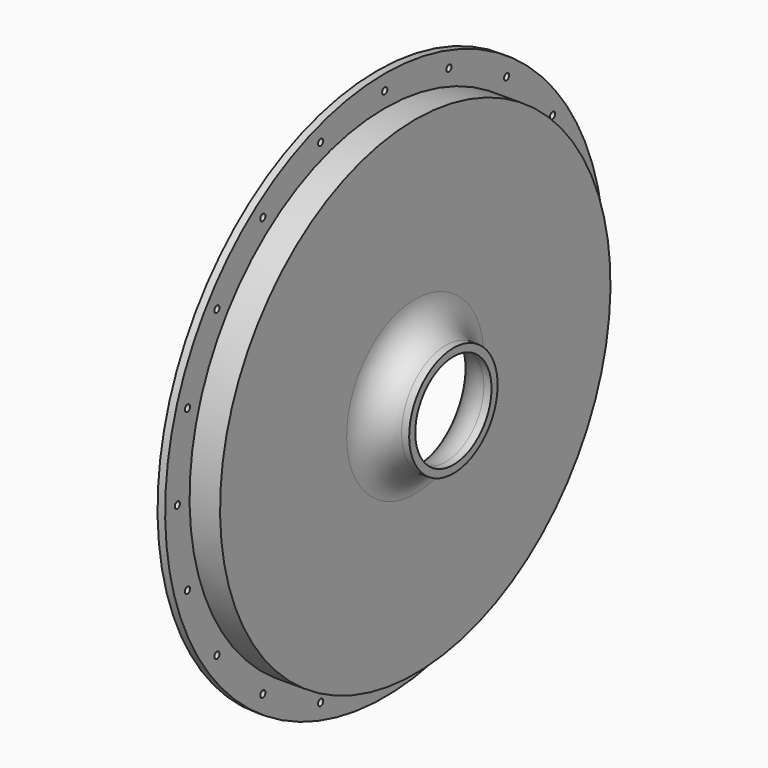
from build123d import *

# Parameters (mm, degrees)
F3_D            = 8.5
F3_COPIES_COUNT = 20


# Not quite as in the source:
# - a pattern or mirror of a feature is missing from the dataset's text; its kind, count and spacing are read off the source's solid


with BuildPart() as f1:
    # F0 (on Front) → F1 (revolve)
    with BuildSketch(Plane.XZ):
        with BuildLine():
            Line((40, 310), (40, 112.5))
            ThreePointArc((40, 112.5), (54.6446609407, 77.1446609407), (90, 62.5))
            Line((90, 62.5), (100, 62.5))
            Line((100, 62.5), (100, 72.5))
            Line((100, 72.5), (90, 72.5))
            ThreePointArc((90, 72.5), (61.7157287525, 84.2157287525), (50, 112.5))
            Line((50, 112.5), (50, 320))
            Line((50, 320), (10, 320))
            Line((10, 320), (10, 360))
            Line((10, 360), (0, 360))
            Line((0, 360), (0, 310))
            Line((0, 310), (40, 310))
        make_face()
    revolve(axis=Axis((50, 0, 0), (1, 0, 0)))

    # F3 (through all)
    with Locations(Plane.YZ.offset(10)):
        with Locations((0, 340)):
            f3 = Hole(F3_D / 2)

    # F3_copies: F3 ×20 about axis
    f3_copies_axis = Axis((0, 0, 0), (1, 0, 0))
    for i in range(1, F3_COPIES_COUNT):
        add(f3.rotate(f3_copies_axis, i * 360 / F3_COPIES_COUNT), mode=Mode.SUBTRACT)


solid = f1.part
